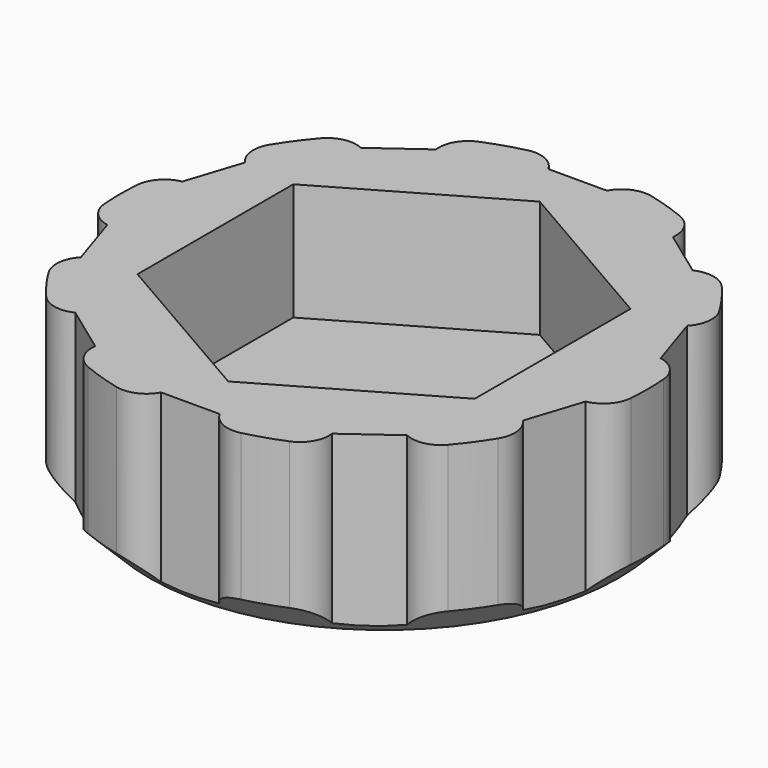
from build123d import *

# Parameters (mm, degrees)
F0_R        = 9
F1_DEPTH    = 4
F2_R        = 9
F3_DEPTH    = 2
F4_SIZE     = 1
F5_W        = 2
F5_H        = 1.5
F6_DEPTH    = 6.001
F7_T1_DEPTH = 10.6633310907


# Not quite as in the source:
# - a fillet or chamfer that OpenCascade refuses, or shapes differently, is made with other operations: its cross-section is extruded or revolved along the edge and cut away or added


with BuildPart() as f1:
    # F0 (on Top) → F1 (new body)
    with BuildSketch(Plane.XY):
        Circle(F0_R)
        Polygon((-5.75, 3.3197640478), (0, 6.6395280957), (5.75, 3.3197640478), (5.75, -3.3197640478), (0, -6.6395280957), (-5.75, -3.3197640478), align=None, mode=Mode.SUBTRACT)
    extrude(amount=F1_DEPTH)

    # F2 (on face) → F3 (join)
    with BuildSketch(Plane(origin=(0, 0, 0), x_dir=(1, 0, 0), z_dir=(0, 0, -1))):
        Circle(F2_R)
    extrude(amount=F3_DEPTH)

    # F4
    f4_edges = [f1.edges().sort_by_distance(p)[0] for p in [
        (-9, 0, -2),
    ]]
    chamfer(f4_edges, length=F4_SIZE)

    # F5 (on face) → F6 (cut, through all)
    with BuildSketch(Plane.XY.offset(4)):
        with Locations((0, 9)):
            Rectangle(F5_W, F5_H)
        Polygon((-4.040211337, 7.2621754559), (-4.9218892155, 8.4757009474), (-6.5399232042, 7.3001304429), (-5.6582453258, 6.0866049513), align=None)
        Polygon((-7.5371992651, 3.5004467199), (-8.9637840395, 3.9639722115), (-9.5818180283, 2.0618591789), (-8.1552332538, 1.5983336873), align=None)
        Polygon((-8.1552332538, -1.5983336873), (-9.5818180283, -2.0618591789), (-8.9637840395, -3.9639722115), (-7.5371992651, -3.5004467199), align=None)
        Polygon((-5.6582453258, -6.0866049513), (-6.5399232042, -7.3001304429), (-4.9218892155, -8.4757009474), (-4.040211337, -7.2621754559), align=None)
        with Locations((0, -9)):
            Rectangle(F5_W, F5_H)
        Polygon((4.040211337, -7.2621754559), (4.9218892155, -8.4757009474), (6.5399232042, -7.3001304429), (5.6582453258, -6.0866049513), align=None)
        Polygon((7.5371992651, -3.5004467199), (8.9637840395, -3.9639722115), (9.5818180283, -2.0618591789), (8.1552332538, -1.5983336873), align=None)
        Polygon((8.1552332538, 1.5983336873), (9.5818180283, 2.0618591789), (8.9637840395, 3.9639722115), (7.5371992651, 3.5004467199), align=None)
        Polygon((5.6582453258, 6.0866049513), (6.5399232042, 7.3001304429), (4.9218892155, 8.4757009474), (4.040211337, 7.2621754559), align=None)
    extrude(amount=-F6_DEPTH, mode=Mode.SUBTRACT)

    # F7: fillet of radius 1 on 20 edges, made by hand

    # F7_s2 → F7_t1 (cut)
    with BuildSketch(Plane.XY.offset(-3.8316655453)):
        with BuildLine():
            ThreePointArc((2.1155025829, 8.7478368081), (1.4729019887, 8.6890401766), (1, 8.25))
            Line((1, 8.25), (1, 8.94427191))
            ThreePointArc((1, 8.94427191), (1.5608445705, 8.8636202664), (2.1155025829, 8.7478368081))
        make_face()
        with BuildLine():
            ThreePointArc((4.040211337, 7.2621754559), (3.9156869325, 7.8953312347), (3.4303719241, 8.3206098612))
            ThreePointArc((3.4303719241, 8.3206098612), (3.9471554914, 8.0882608469), (4.4482941268, 7.8238532298))
            Line((4.4482941268, 7.8238532298), (4.040211337, 7.2621754559))
        make_face()
        with BuildLine():
            ThreePointArc((6.8533270065, 5.8336874224), (6.2988924123, 6.1638311007), (5.6582453258, 6.0866049513))
            Line((5.6582453258, 6.0866049513), (6.0663281156, 6.6482827252))
            ThreePointArc((6.0663281156, 6.6482827252), (6.4726550576, 6.2533780075), (6.8533270065, 5.8336874224))
        make_face()
        with BuildLine():
            ThreePointArc((7.5371992651, 3.5004467199), (7.8086165348, 4.0858741136), (7.6659609501, 4.7151927544))
            ThreePointArc((7.6659609501, 4.7151927544), (7.9474763144, 4.2234606937), (8.1974910891, 3.7149885388))
            Line((8.1974910891, 3.7149885388), (7.5371992651, 3.5004467199))
        make_face()
        with BuildLine():
            ThreePointArc((8.9734134496, 0.691267721), (8.7189200259, 1.2842480452), (8.1552332538, 1.5983336873))
            Line((8.1552332538, 1.5983336873), (8.8155250779, 1.8128755062))
            ThreePointArc((8.8155250779, 1.8128755062), (8.9121313102, 1.2545578943), (8.9734134496, 0.691267721))
        make_face()
        with BuildLine():
            ThreePointArc((8.9734134496, -0.691267721), (8.7189200259, -1.2842480452), (8.1552332538, -1.5983336873))
            Line((8.1552332538, -1.5983336873), (8.8155250779, -1.8128755062))
            ThreePointArc((8.8155250779, -1.8128755062), (8.9121313102, -1.2545578943), (8.9734134496, -0.691267721))
        make_face()
        with BuildLine():
            ThreePointArc((7.6659609501, -4.7151927544), (7.8086165348, -4.0858741136), (7.5371992651, -3.5004467199))
            Line((7.5371992651, -3.5004467199), (8.1974910891, -3.7149885388))
            ThreePointArc((8.1974910891, -3.7149885388), (7.9474763144, -4.2234606937), (7.6659609501, -4.7151927544))
        make_face()
        with BuildLine():
            ThreePointArc((5.6582453258, -6.0866049513), (6.2988924123, -6.1638311007), (6.8533270065, -5.8336874224))
            ThreePointArc((6.8533270065, -5.8336874224), (6.4726550576, -6.2533780075), (6.0663281156, -6.6482827252))
            Line((6.0663281156, -6.6482827252), (5.6582453258, -6.0866049513))
        make_face()
        with BuildLine():
            ThreePointArc((3.4303719241, -8.3206098612), (3.9156869325, -7.8953312347), (4.040211337, -7.2621754559))
            Line((4.040211337, -7.2621754559), (4.4482941268, -7.8238532298))
            ThreePointArc((4.4482941268, -7.8238532298), (3.9471554914, -8.0882608469), (3.4303719241, -8.3206098612))
        make_face()
        with BuildLine():
            ThreePointArc((1, -8.25), (1.4729019887, -8.6890401766), (2.1155025829, -8.7478368081))
            ThreePointArc((2.1155025829, -8.7478368081), (1.5608445705, -8.8636202664), (1, -8.94427191))
            Line((1, -8.94427191), (1, -8.25))
        make_face()
        with BuildLine():
            ThreePointArc((-2.1155025829, -8.7478368081), (-1.4729019887, -8.6890401766), (-1, -8.25))
            Line((-1, -8.25), (-1, -8.94427191))
            ThreePointArc((-1, -8.94427191), (-1.5608445705, -8.8636202664), (-2.1155025829, -8.7478368081))
        make_face()
        with BuildLine():
            ThreePointArc((-4.040211337, -7.2621754559), (-3.9156869325, -7.8953312347), (-3.4303719241, -8.3206098612))
            ThreePointArc((-3.4303719241, -8.3206098612), (-3.9471554914, -8.0882608469), (-4.4482941268, -7.8238532298))
            Line((-4.4482941268, -7.8238532298), (-4.040211337, -7.2621754559))
        make_face()
        with BuildLine():
            ThreePointArc((-6.8533270065, -5.8336874224), (-6.2988924123, -6.1638311007), (-5.6582453258, -6.0866049513))
            Line((-5.6582453258, -6.0866049513), (-6.0663281156, -6.6482827252))
            ThreePointArc((-6.0663281156, -6.6482827252), (-6.4726550576, -6.2533780075), (-6.8533270065, -5.8336874224))
        make_face()
        with BuildLine():
            ThreePointArc((-7.5371992651, -3.5004467199), (-7.8086165348, -4.0858741136), (-7.6659609501, -4.7151927544))
            ThreePointArc((-7.6659609501, -4.7151927544), (-7.9474763144, -4.2234606937), (-8.1974910891, -3.7149885388))
            Line((-8.1974910891, -3.7149885388), (-7.5371992651, -3.5004467199))
        make_face()
        with BuildLine():
            ThreePointArc((-8.9734134496, -0.691267721), (-8.7189200259, -1.2842480452), (-8.1552332538, -1.5983336873))
            Line((-8.1552332538, -1.5983336873), (-8.8155250779, -1.8128755062))
            ThreePointArc((-8.8155250779, -1.8128755062), (-8.9121313102, -1.2545578943), (-8.9734134496, -0.691267721))
        make_face()
        with BuildLine():
            ThreePointArc((-8.1552332538, 1.5983336873), (-8.7189200259, 1.2842480452), (-8.9734134496, 0.691267721))
            ThreePointArc((-8.9734134496, 0.691267721), (-8.9121313102, 1.2545578943), (-8.8155250779, 1.8128755062))
            Line((-8.8155250779, 1.8128755062), (-8.1552332538, 1.5983336873))
        make_face()
        with BuildLine():
            ThreePointArc((-7.6659609501, 4.7151927544), (-7.8086165348, 4.0858741136), (-7.5371992651, 3.5004467199))
            Line((-7.5371992651, 3.5004467199), (-8.1974910891, 3.7149885388))
            ThreePointArc((-8.1974910891, 3.7149885388), (-7.9474763144, 4.2234606937), (-7.6659609501, 4.7151927544))
        make_face()
        with BuildLine():
            ThreePointArc((-5.6582453258, 6.0866049513), (-6.2988924123, 6.1638311007), (-6.8533270065, 5.8336874224))
            ThreePointArc((-6.8533270065, 5.8336874224), (-6.4726550576, 6.2533780075), (-6.0663281156, 6.6482827252))
            Line((-6.0663281156, 6.6482827252), (-5.6582453258, 6.0866049513))
        make_face()
        with BuildLine():
            ThreePointArc((-3.4303719241, 8.3206098612), (-3.9156869325, 7.8953312347), (-4.040211337, 7.2621754559))
            Line((-4.040211337, 7.2621754559), (-4.4482941268, 7.8238532298))
            ThreePointArc((-4.4482941268, 7.8238532298), (-3.9471554914, 8.0882608469), (-3.4303719241, 8.3206098612))
        make_face()
        with BuildLine():
            ThreePointArc((-1, 8.25), (-1.4729019887, 8.6890401766), (-2.1155025829, 8.7478368081))
            ThreePointArc((-2.1155025829, 8.7478368081), (-1.5608445705, 8.8636202664), (-1, 8.94427191))
            Line((-1, 8.94427191), (-1, 8.25))
        make_face()
    extrude(amount=F7_T1_DEPTH, mode=Mode.SUBTRACT)


solid = f1.part
